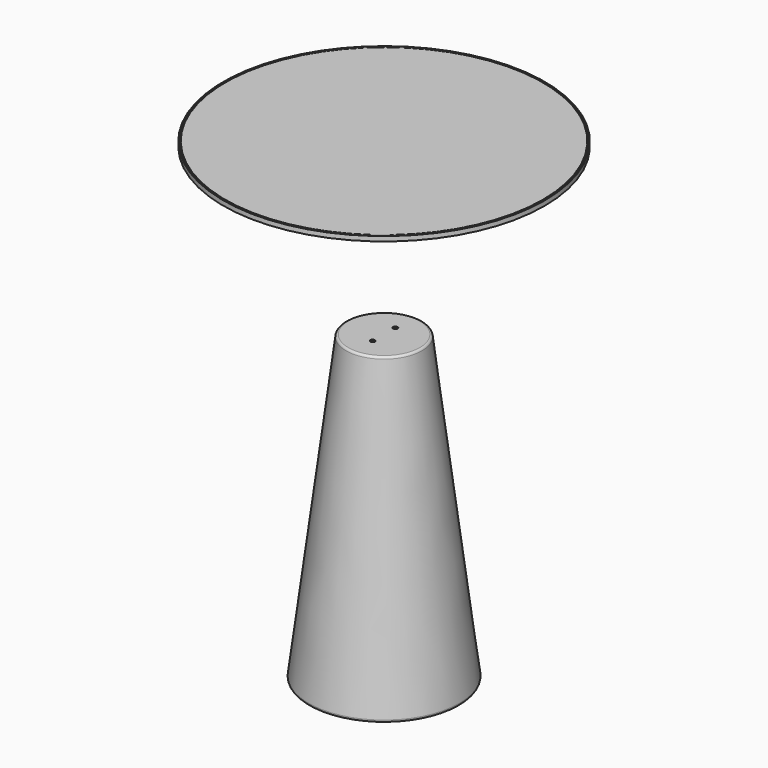
from build123d import *

# Parameters (mm, degrees)
F2_T      = -1.778
F3_T      = -1.778
F4_R      = 213.32825
F5_DEPTH  = 6.35
F8_D      = 6.096
F8_DEPTH  = 5.08
F8_TIP    = 1.8314231668
F10_D     = 6.096
F10_DEPTH = 5.08
F10_TIP   = 1.8314231668


# Not quite as in the source:
# - a fillet or chamfer that OpenCascade refuses, or shapes differently, is made with other operations: its cross-section is extruded or revolved along the edge and cut away or added


with BuildPart() as f1:
    # F0 (on Front) → F1 (revolve)
    with BuildSketch(Plane.XZ):
        Polygon((215.9, 311.15), (215.9, 317.5), (0, 317.5), (0, 241.3), (25.4, 241.3), (28.575, 241.3), align=None)
    revolve(axis=Axis((0, 0, 279.4), (0, 0, -1)))

    # F3
    f3_openings = [f1.faces().sort_by_distance(p)[0] for p in [
        (0, 0, 317.5),
    ]]
    offset(amount=F3_T, openings=f3_openings)

    # F8
    with Locations(Plane(origin=(0, 0, 241.3), x_dir=(1, 0, 0), z_dir=(0, 0, -1))):
        with Locations((-0.2177452552, 15.1099245586), (-0.2177452552, -16.6400754414)):
            Hole(F8_D / 2, depth=F8_DEPTH)
            with Locations((0, 0, -(F8_DEPTH + F8_TIP / 2))):  # 118° drill point
                Cone(0, F8_D / 2, F8_TIP, mode=Mode.SUBTRACT)


with BuildPart() as f1b:
    # F0 (on Front) → F1, piece 2 (revolve)
    with BuildSketch(Plane.XZ):
        Polygon((0, 88.9), (0, -317.5), (101.6, -317.5), (50.8, 88.9), (38.1, 88.9), align=None)
    revolve(axis=Axis((0, 0, 279.4), (0, 0, -1)))

    # F2
    f2_openings = [f1b.faces().sort_by_distance(p)[0] for p in [
        (0, 0, -317.5),
    ]]
    offset(amount=F2_T, openings=f2_openings)

    # F6: fillet of radius 3.175 on 2 edges, made by hand

    # F6_s1 → F6_t2 (revolve, cut)
    with BuildSketch(Plane.XZ):
        with BuildLine():
            ThreePointArc((51.1481767954, 86.1178105398), (50.0983895944, 88.1052282082), (47.9961089334, 88.9004))
            Line((47.9961089334, 88.9004), (47.9961089334, 89.2180597943))
            ThreePointArc((47.9961089334, 89.2180597943), (49.3980544667, 89.2176597943), (50.8, 89.2176597943))
            Line((50.8, 89.2176597943), (51.1152067862, 88.9394008483))
            ThreePointArc((51.1152067862, 88.9394008483), (51.2890967283, 87.5482813112), (51.4633835816, 86.1572113881))
            Line((51.4633835816, 86.1572113881), (51.1481767954, 86.1178105398))
        make_face()
    revolve(axis=Axis((0, 0, 88.9), (0, 0, -1)), mode=Mode.SUBTRACT)

    # F6_s3 → F6_t4 (revolve, cut)
    with BuildSketch(Plane.XZ):
        with BuildLine():
            ThreePointArc((101.2191288957, -314.4498062625), (100.9503066223, -316.1769576353), (99.8083824609, -317.5003345615))
            Line((99.8083824609, -317.5003345615), (99.9824734041, -317.7659916931))
            ThreePointArc((99.9824734041, -317.7659916931), (100.7041912305, -317.8176182741), (101.6, -317.8176182741))
            Line((101.6, -317.8176182741), (101.9151655866, -317.4606043017))
            ThreePointArc((101.9151655866, -317.4606043017), (101.7245315789, -315.9355322399), (101.5342944823, -314.4104105642))
            Line((101.5342944823, -314.4104105642), (101.2191288957, -314.4498062625))
        make_face()
    revolve(axis=Axis((0, 0, -317.5), (0, 0, -1)), mode=Mode.SUBTRACT)

    # F10
    with Locations(Plane.XY.offset(88.9)):
        with Locations((-0.0706888968, -18.9808944534), (-0.0706888968, 19.1191055466)):
            Hole(F10_D / 2, depth=F10_DEPTH)
            with Locations((0, 0, -(F10_DEPTH + F10_TIP / 2))):  # 118° drill point
                Cone(0, F10_D / 2, F10_TIP, mode=Mode.SUBTRACT)


with BuildPart() as f5:
    # F4 (on face) → F5 (new body)
    with BuildSketch(Plane.XY.offset(317.5)):
        Circle(F4_R)
    extrude(amount=-F5_DEPTH)


solid = Compound([f1.part, f1b.part, f5.part])
